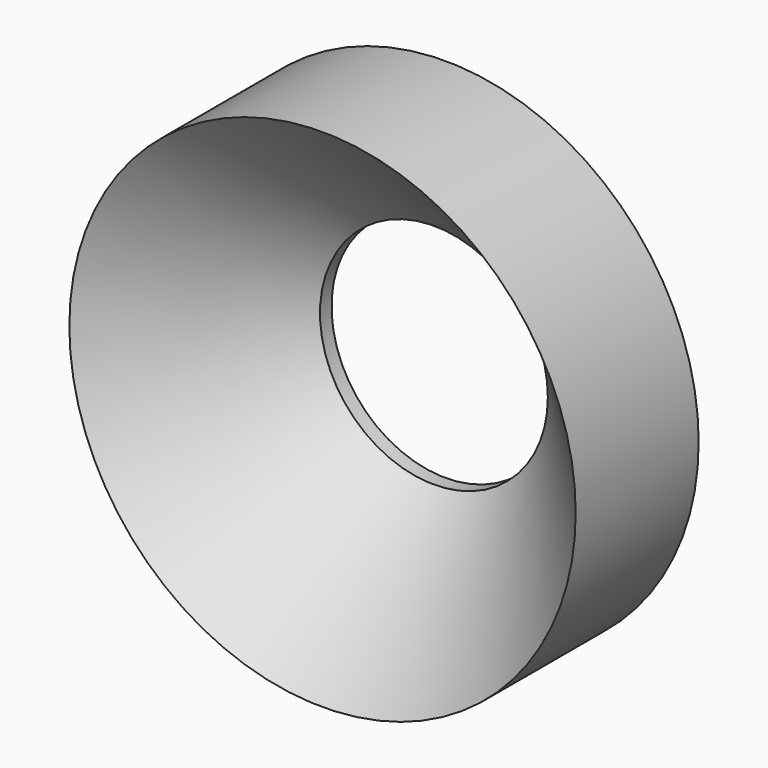
from build123d import *

# Parameters (mm, degrees)
F0_R     = 3.5
F0_R_2   = 1.575
F1_DEPTH = 2.2
F2_DEPTH = 4


# Not quite as in the source:
# - a fillet or chamfer that OpenCascade refuses, or shapes differently, is made with other operations: its cross-section is extruded or revolved along the edge and cut away or added


with BuildPart() as f1:
    # F0 (on Front) → F1 (new body)
    with BuildSketch(Plane.XZ):
        Circle(F0_R)
        Circle(F0_R_2, mode=Mode.SUBTRACT)
        Circle(F0_R_2)
    extrude(amount=F1_DEPTH)

    # F0 (on Front) → F2 (cut)
    with BuildSketch(Plane.XZ):
        Circle(F0_R_2)
    extrude(amount=F2_DEPTH, mode=Mode.SUBTRACT)

    # F3: chamfer of 2 on 1 edges, made by hand

    # F3_s1 → F3_t2 (revolve, cut)
    with BuildSketch(Plane.XY):
        Polygon((3.575, -2.2), (1.575, -0.2), (1.575, -2.2), align=None)
    revolve(axis=Axis((0, -2.2, 0), (0, 1, 0)), mode=Mode.SUBTRACT)


solid = f1.part
